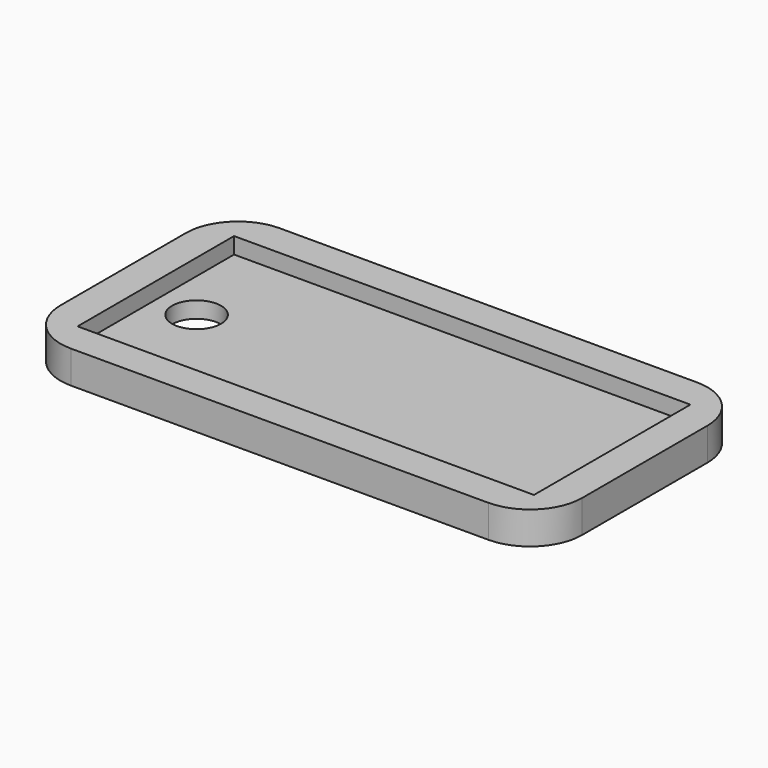
from build123d import *

# Parameters (mm, degrees)
F0_W     = 44.45
F0_H     = 19.05
F0_R     = 2.38125
F1_DEPTH = 1.5875
F0_W_2   = 50.8
F0_H_2   = 25.4
F2_DEPTH = 3.175
F3_R     = 5.08


# Not quite as in the source:
# - a length typed as a fraction of an inch, garbled in the dataset ("3 / 203.2 mm" for 3/8 in), is restored


with BuildPart() as f1:
    # F0 (on Top) → F1 (new body)
    with BuildSketch(Plane.XY):
        with Locations((25.4, 12.7)):
            Rectangle(F0_W, F0_H)
        with Locations((7.14375, 12.7)):
            Circle(F0_R, mode=Mode.SUBTRACT)
    extrude(amount=F1_DEPTH)

    # F0 (on Top) → F2 (join)
    with BuildSketch(Plane.XY):
        with Locations((25.4, 12.7)):
            Rectangle(F0_W_2, F0_H_2)
        with Locations((25.4, 12.7)):
            Rectangle(F0_W, F0_H, mode=Mode.SUBTRACT)
    extrude(amount=F2_DEPTH)

    # F3
    f3_edges = [f1.edges().sort_by_distance(p)[0] for p in [
        (50.8, 0, 1.5875),
        (50.8, 25.4, 1.5875),
        (0, 0, 1.5875),
        (0, 25.4, 1.5875),
    ]]
    fillet(f3_edges, radius=F3_R)


solid = f1.part
